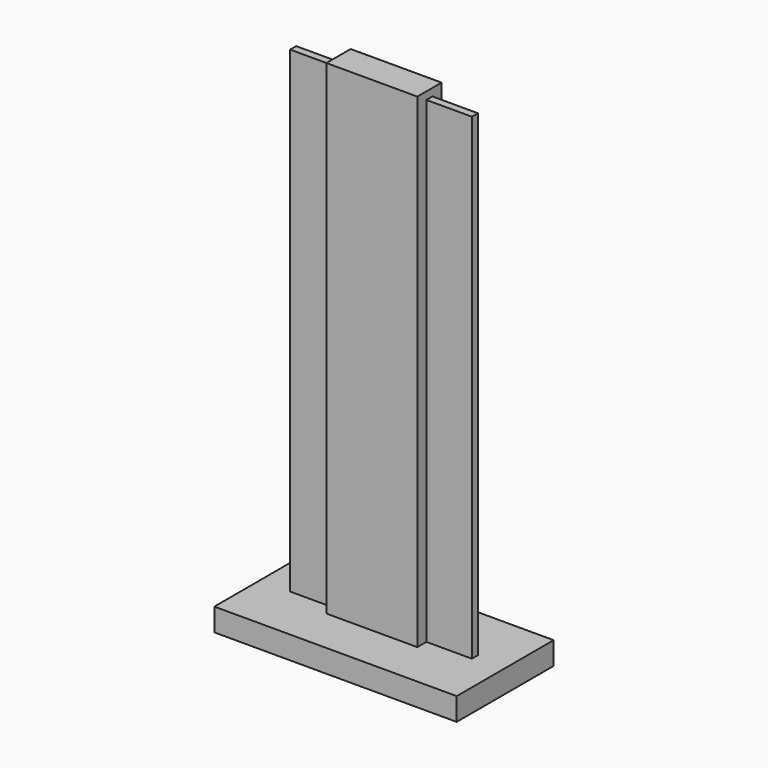
from build123d import *

# Parameters (mm, degrees)
F0_W     = 203.2
F0_H     = 101.6
F0_W_2   = 76.2
F0_H_2   = 9.525
F0_W_3   = 38.1
F0_H_3   = 6.35
F1_DEPTH = 19.05
F2_DEPTH = 406.4
F3_DEPTH = 400.05
F4_W     = 76.2
F4_H     = 9.525
F4_H_2   = 6.35
F5_DEPTH = 6.35


with BuildPart() as f1:
    # F0 (on Top) → F1 (new body)
    with BuildSketch(Plane.XY):
        Rectangle(F0_W, F0_H)
        Polygon((-38.1, 12.7), (38.1, 12.7), (38.1, 3.175), (76.2, 3.175), (76.2, -3.175), (38.1, -3.175), (38.1, -12.7), (-38.1, -12.7), (-38.1, -3.175), (-76.2, -3.175), (-76.2, 3.175), (-38.1, 3.175), align=None, mode=Mode.SUBTRACT)
        with Locations((0, 7.9375)):
            Rectangle(F0_W_2, F0_H_2)
        with Locations((57.15, 0)):
            Rectangle(F0_W_3, F0_H_3)
        Rectangle(F0_W_2, F0_H_3)
        with Locations((0, -7.9375)):
            Rectangle(F0_W_2, F0_H_2)
        with Locations((-57.15, 0)):
            Rectangle(F0_W_3, F0_H_3)
    extrude(amount=-F1_DEPTH)


with BuildPart() as f2:
    # F0 (on Top) → F2 (new body)
    with BuildSketch(Plane.XY):
        with Locations((0, 7.9375)):
            Rectangle(F0_W_2, F0_H_2)
    extrude(amount=F2_DEPTH)



with BuildPart() as f2b:
    # F0 (on Top) → F2, piece 2 (new body)
    with BuildSketch(Plane.XY):
        with Locations((0, -7.9375)):
            Rectangle(F0_W_2, F0_H_2)
    extrude(amount=F2_DEPTH)


with BuildPart() as f3:
    # F0 (on Top) → F3 (new body)
    with BuildSketch(Plane.XY):
        with Locations((57.15, 0)):
            Rectangle(F0_W_3, F0_H_3)
        Rectangle(F0_W_2, F0_H_3)
        with Locations((-57.15, 0)):
            Rectangle(F0_W_3, F0_H_3)
    extrude(amount=F3_DEPTH)


with BuildPart() as f2_1:
    add(f2.part)

    add(f2b.part)  # F5 merges F2b
    # F4 (on face) → F5 (join)
    with BuildSketch(Plane.XY.offset(406.4)):
        with Locations((0, 7.9375)):
            Rectangle(F4_W, F4_H)
        Rectangle(F4_W, F4_H_2)
    extrude(amount=-F5_DEPTH)


solid = Compound([f1.part, f3.part, f2_1.part])
